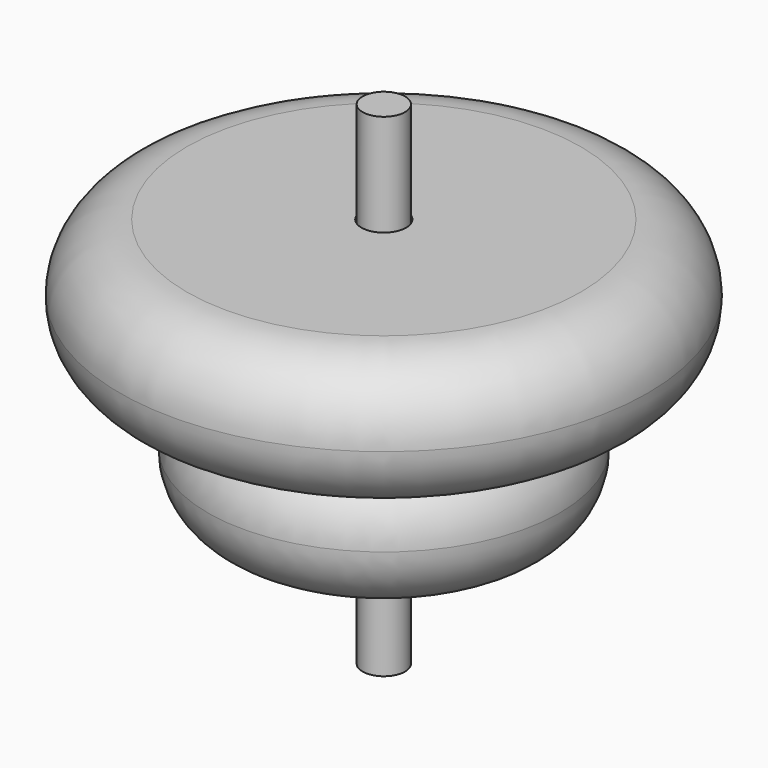
from build123d import *

# Parameters (mm, degrees)
F0_R     = 100
F0_R_2   = 12.7
F1_DEPTH = 76.2
F2_R     = 150
F2_R_2   = 100
F2_R_3   = 12.7
F3_DEPTH = 76.2
F4_R     = 38.09999
F5_R     = 38.09999
F0_R_3   = 12.065
F6_DEPTH = 210
F7_DEPTH = 69.85


# Not quite as in the source:
# - a fillet or chamfer is up to 0.001 mm smaller than in the source, because OpenCascade refuses the exact size


with BuildPart() as f1:
    # F0 (on Top) → F1 (new body)
    with BuildSketch(Plane.XY):
        Circle(F0_R)
        Circle(F0_R_2, mode=Mode.SUBTRACT)
    extrude(amount=F1_DEPTH)

    # F4 (radius 38.1 in the source; OpenCascade refuses exactly that, so slightly less here)
    f4_edges = [f1.edges().sort_by_distance(p)[0] for p in [
        (100, 0, 38.1),
        (-100, 0, 0),
        (-100, 0, 76.2),
    ]]
    fillet(f4_edges, radius=F4_R)


with BuildPart() as f3:
    # F2 (on face) → F3 (new body)
    with BuildSketch(Plane.XY.offset(76.2)):
        Circle(F2_R)
        Circle(F2_R_2, mode=Mode.SUBTRACT)
        Circle(F2_R_2)
        Circle(F2_R_3, mode=Mode.SUBTRACT)
    extrude(amount=F3_DEPTH)

    # F5 (radius 38.1 in the source; OpenCascade refuses exactly that, so slightly less here)
    f5_edges = [f3.edges().sort_by_distance(p)[0] for p in [
        (150, 0, 114.3),
        (-150, 0, 76.2),
        (-150, 0, 152.4),
    ]]
    fillet(f5_edges, radius=F5_R)


with BuildPart() as f6:
    # F0 (on Top) → F6 (new body)
    with BuildSketch(Plane.XY):
        Circle(F0_R_3)
    extrude(amount=F6_DEPTH)

    # F7 (add): a face of the model
    f7_faces = [f6.faces().sort_by_distance(p)[0] for p in [
        (0, 0, 0),
    ]]
    extrude(f7_faces, amount=F7_DEPTH)


solid = Compound([f1.part, f3.part, f6.part])
